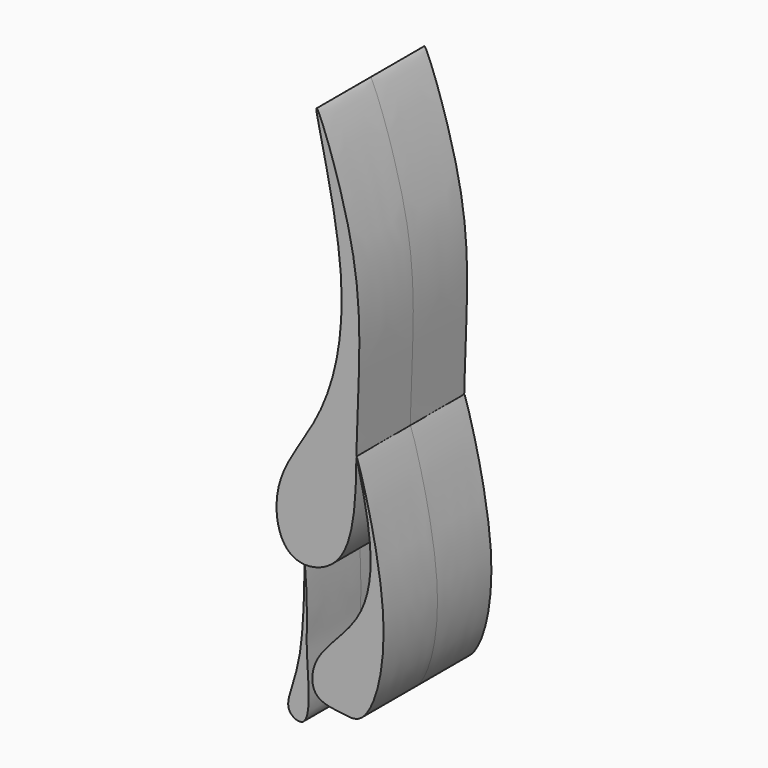
from build123d import *

# Parameters (mm, degrees)
F1_DEPTH = 12.7
F3_DEPTH = 12.7


with BuildPart() as f1:
    # F0 (on Front) → F1 (new body, symmetric)
    with BuildSketch(Plane.XZ):
        with BuildLine():
            add(Edge.make_bspline(
                [(0, 26.208980009), (0.4496034082, 26.4013627069), (9.7793291876, 1.7288186438), (6.96636093, -22.7817814425), (7.97554798, -48.7894146057), (-6.631042909, -51.9651575575), (-8.9877715907, -37.4658728522), (1.9451011553, -24.9977853921), (7.4506672672, -1.2041408772), (-0.479166736, 26.003947334), (0, 26.208980009)],
                knots=[0, 0, 0, 0, 0.1319413383, 0.287922325, 0.4225918184, 0.5071990681, 0.5995330288, 0.7115902774, 0.8593829601, 1, 1, 1, 1], degree=3))
        make_face()
    extrude(amount=F1_DEPTH, both=True)

    # F2 (on Front) → F3, piece 2 (join, symmetric)
    with BuildSketch(Plane.XZ):
        with BuildLine():
            add(Edge.make_bspline(
                [(-2.2445206996, -49.9906949699), (-2.146966117, -49.9755461744), (-1.5658084612, -59.1540168318), (-2.2038087531, -63.6951865693), (-0.5449143401, -78.1553471452), (-6.9904425987, -75.2684583522), (-1.9035827183, -67.5018821609), (-2.3873679627, -50.0128770542), (-2.2445206996, -49.9906949699)],
                knots=[0, 0, 0, 0, 0.1569111411, 0.3114384904, 0.5027003582, 0.596953546, 0.7702380917, 1, 1, 1, 1], degree=3))
        make_face()
    extrude(amount=F3_DEPTH, both=True)


with BuildPart() as f3:
    # F2 (on Front) → F3 (new body, symmetric)
    with BuildSketch(Plane.XZ):
        with BuildLine():
            add(Edge.make_bspline(
                [(7.5498661026, -29.0960036218), (7.7355192605, -29.1867694531), (15.597323601, -55.0030027864), (9.9204959865, -73.4927330999), (4.8211330884, -72.5665794361), (-1.1424232648, -72.0547992182), (-0.9824759617, -64.2412375162), (9.1665548284, -56.6730175797), (11.3603986941, -43.283342748), (7.4186988127, -29.0318759321), (7.5498661026, -29.0960036218)],
                knots=[0, 0, 0, 0, 0.1880700499, 0.3499124619, 0.4220650925, 0.5053183116, 0.5942429114, 0.7222081306, 0.8671251325, 1, 1, 1, 1], degree=3))
        make_face()
    extrude(amount=F3_DEPTH, both=True)


solid = Compound([f1.part, f3.part])
